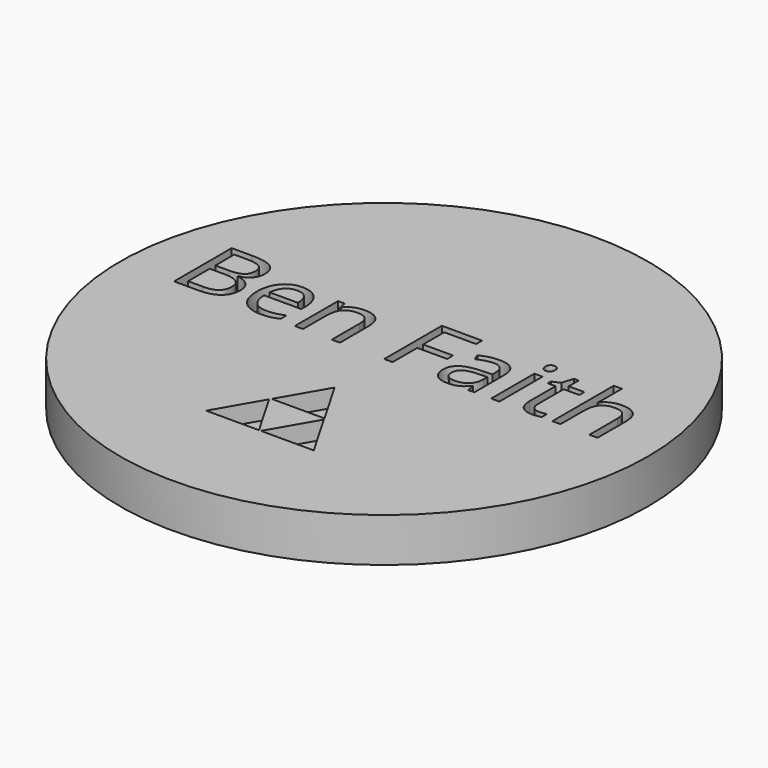
from build123d import *

# Parameters (mm, degrees)
F0_R         = 38.1
F1_DEPTH     = 6.35
F2_TEXT_SIZE = 14.5678746819
F3_DEPTH     = 2.54
F5_DEPTH     = 2.54


# Not quite as in the source:
# - ends of sketch curves that miss each other by under 0.0002 mm in the source are joined
# - Text() gives the source's letters only with a copy of the font that has no kerning and outlines rounded to 1/6400 em; it was checked with that copy


with BuildPart() as f1:
    # F0 (on Top) → F1 (new body)
    with BuildSketch(Plane.XY):
        Circle(F0_R)
    extrude(amount=F1_DEPTH)

    # F2 (on face) → F3 (cut)
    with BuildSketch(Plane.XY.offset(6.35)):
        with Locations((-31.75, 0)):
            Text('Ben Faith', F2_TEXT_SIZE, font='Open Sans', text_align=(TextAlign.LEFT, TextAlign.BOTTOM))
    extrude(amount=-F3_DEPTH, mode=Mode.SUBTRACT)

    # F4 (on face) → F5 (cut)
    with BuildSketch(Plane.XY.offset(6.35)):
        Polygon((3.9370004721, -15.7789066843), (0.127, -22.3780199885), (7.747, -22.3780199885), align=None)
        Polygon((3.8100000926, -15.5249073415), (9.26e-08, -8.9257937647), (-3.8099999074, -15.5249073415), align=None)
        Polygon((-0.1577181855, -22.3780190587), (-3.9677185187, -15.7789056742), (-7.7777185187, -22.3780192511), align=None)
    extrude(amount=-F5_DEPTH, mode=Mode.SUBTRACT)


solid = f1.part
